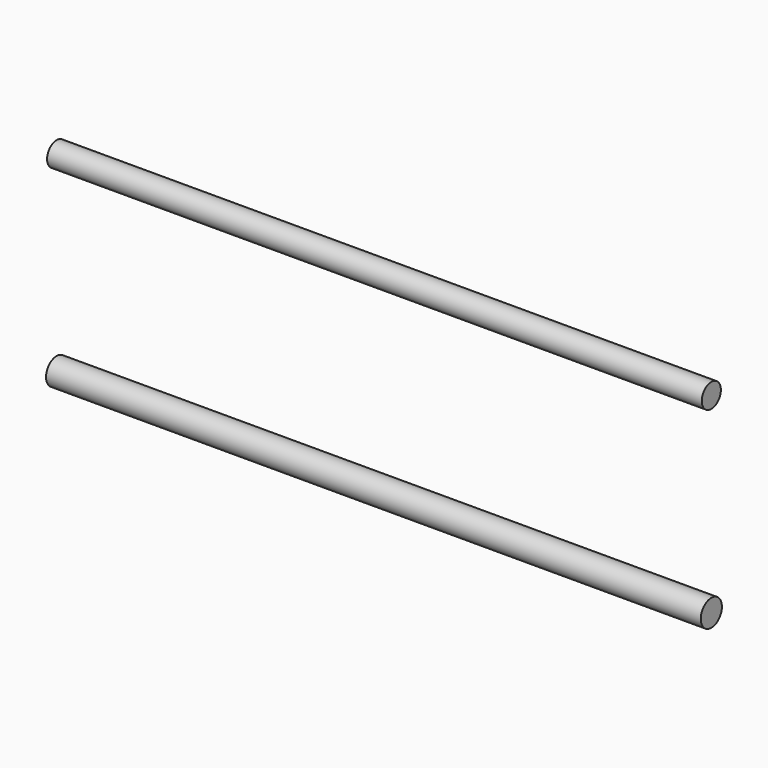
from build123d import *

# Parameters (mm, degrees)
F3_R          = 0.9251736669
F4_DEPTH      = 25.4
F4_DEPTH_BACK = 25.4
F3_R_2        = 1.0263908893


# Not quite as in the source:
# - a feature of the source that left no trace in its solid (it failed there, or was rolled back) is left out
# - the program builds the solid bodies; features that only make, move or delete a surface that nothing else refers to are left out


with BuildPart() as f4:
    # F3 (on Right) → F4 (new body, two sides)
    with BuildSketch(Plane.YZ) as f4_sk:
        with Locations((-48.2449010015, 17.1755533665)):
            Circle(F3_R)
    extrude(amount=F4_DEPTH)
    extrude(f4_sk.sketch, amount=-F4_DEPTH_BACK)


with BuildPart() as f4b:
    # F3 (on Right) → F4, piece 2 (new body, two sides)
    with BuildSketch(Plane.YZ) as f4_2_sk:
        with Locations((-48.2449010015, 2.3263529874)):
            Circle(F3_R_2)
    extrude(amount=F4_DEPTH)
    extrude(f4_2_sk.sketch, amount=-F4_DEPTH_BACK)


solid = Compound([f4.part, f4b.part])
